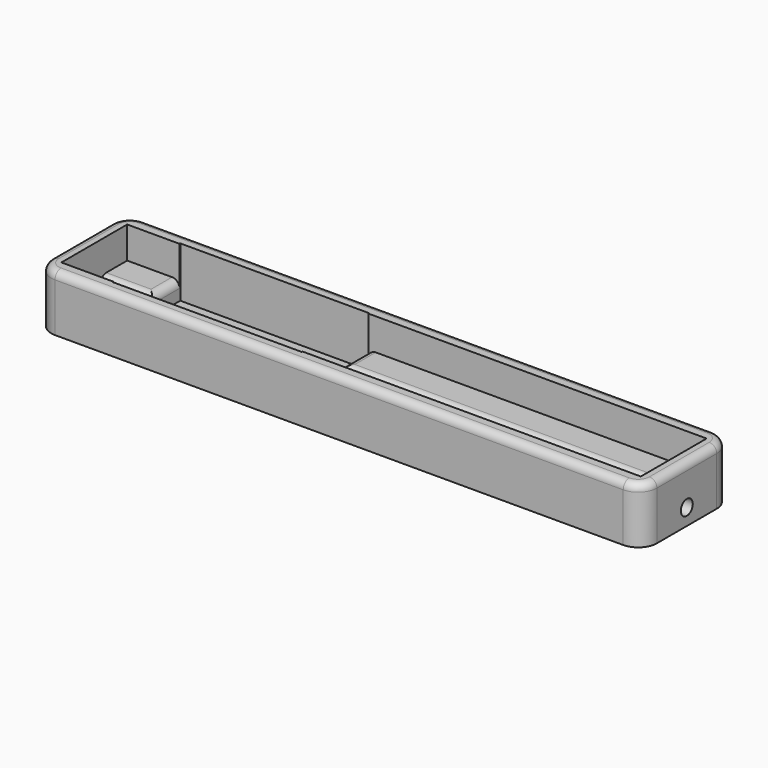
from build123d import *

# Parameters (mm, degrees)
F0_W         = 50.5
F0_H         = 9
F0_H_2       = 2
F0_W_2       = 12.75
F0_H_3       = 0.25
F0_W_3       = 1.2480659857
F1_DEPTH     = 1.5
F0_W_4       = 77.7519340143
F2_DEPTH     = 6.5
F3_DEPTH     = 15
F4_R         = 2
F5_DEPTH     = 162.001
F6_R         = 2
F7_T1_DEPTH  = 27.5
F7_T4_ANGLE  = 90
F7_T6_ANGLE  = 90
F7_T8_ANGLE  = 90
F7_T10_ANGLE = 90


# Not quite as in the source:
# - a fillet or chamfer that OpenCascade refuses, or shapes differently, is made with other operations: its cross-section is extruded or revolved along the edge and cut away or added


with BuildPart() as f1:
    # F0 (on Top) → F1 (new body)
    with BuildSketch(Plane.XY):
        with Locations((8.0849453807, 6.5)):
            Rectangle(F0_W, F0_H)
        with Locations((8.0849453807, 1)):
            Rectangle(F0_W, F0_H_2)
        with Locations((8.0849453807, -1)):
            Rectangle(F0_W, F0_H_2)
        with Locations((-23.5400546193, -1)):
            Rectangle(F0_W_2, F0_H_2)
        with Locations((-23.5400546193, 1)):
            Rectangle(F0_W_2, F0_H_2)
        with Locations((39.7099453807, 1)):
            Rectangle(F0_W_2, F0_H_2)
        with Locations((39.7099453807, -1)):
            Rectangle(F0_W_2, F0_H_2)
        Polygon((46.0849453807, 2), (46.0849453807, 0), (46.0849453807, -2), (123.8368793949, -2), (123.8368793949, 2), align=None)
        with Locations((8.0849453807, -6.5)):
            Rectangle(F0_W, F0_H)
        with Locations((8.0849453807, 11.125)):
            Rectangle(F0_W, F0_H_3)
        with Locations((8.0849453807, -11.125)):
            Rectangle(F0_W, F0_H_3)
        with Locations((-30.5390876122, -1)):
            Rectangle(F0_W_3, F0_H_2)
        with Locations((-30.5390876122, 1)):
            Rectangle(F0_W_3, F0_H_2)
    extrude(amount=F1_DEPTH)

    # F0 (on Top) → F2 (join)
    with BuildSketch(Plane.XY):
        with Locations((-23.5400546193, 6.5)):
            Rectangle(F0_W_2, F0_H)
        with Locations((-30.5390876122, 6.5)):
            Rectangle(F0_W_3, F0_H)
        with Locations((-23.5400546193, -6.5)):
            Rectangle(F0_W_2, F0_H)
        with Locations((-30.5390876122, -6.5)):
            Rectangle(F0_W_3, F0_H)
        with Locations((39.7099453807, -6.5)):
            Rectangle(F0_W_2, F0_H)
        with Locations((39.7099453807, 6.5)):
            Rectangle(F0_W_2, F0_H)
        with Locations((84.9609123878, 6.5)):
            Rectangle(F0_W_4, F0_H)
        with Locations((84.9609123878, -6.5)):
            Rectangle(F0_W_4, F0_H)
    extrude(amount=F2_DEPTH)

    # F0 (on Top) → F3 (join)
    with BuildSketch(Plane.XY):
        Polygon((127.3368793949, -15), (127.3368793949, 15), (-34.6631206051, 15), (-34.6631206051, 0), (-34.6631206051, -15), align=None)
        Polygon((-31.1631206051, -2), (-31.1631206051, 0), (-31.1631206051, 2), (-31.1631206051, 11), (-29.9150546193, 11), (-17.1650546193, 11), (-17.1650546193, 11.25), (33.3349453807, 11.25), (33.3349453807, 11), (46.0849453807, 11), (123.8368793949, 11), (123.8368793949, 2), (123.8368793949, -2), (123.8368793949, -11), (46.0849453807, -11), (33.3349453807, -11), (33.3349453807, -11.25), (-17.1650546193, -11.25), (-17.1650546193, -11), (-29.9150546193, -11), (-31.1631206051, -11), align=None, mode=Mode.SUBTRACT)
    extrude(amount=F3_DEPTH)

    # F4 (on face) → F5 (cut, through all)
    with BuildSketch(Plane.YZ.offset(127.3368793949)):
        with Locations((0, 4.3932246044)):
            Circle(F4_R)
    extrude(amount=-F5_DEPTH, mode=Mode.SUBTRACT)

    # F6
    f6_edges = [f1.edges().sort_by_distance(p)[0] for p in [
        (-24.164088, -2, 6.5),
        (-24.164088, 2, 6.5),
        (-17.165055, -6.5, 6.5),
        (-17.165055, 6.5, 6.5),
        (33.334945, 6.5, 6.5),
        (33.334945, -6.5, 6.5),
        (78.585912, -2, 6.5),
        (78.585912, 2, 6.5),
        (46.336879, 15, 15),
        (-34.663121, 0, 15),
        (46.336879, -15, 15),
        (127.336879, 0, 15),
    ]]
    fillet(f6_edges, radius=F6_R)

    # F7: fillet of radius 5 on 4 edges, made by hand

    # F7_s2 → F7_t1 (cut)
    with BuildSketch(Plane.XY.offset(-12.5)):
        with BuildLine():
            ThreePointArc((-29.6631206051, 15), (-33.198654511, 13.5355339059), (-34.6631206051, 10))
            Line((-34.6631206051, 10), (-34.6631206051, 15))
            Line((-34.6631206051, 15), (-29.6631206051, 15))
        make_face()
        with BuildLine():
            ThreePointArc((-34.6631206051, -10), (-33.198654511, -13.5355339059), (-29.6631206051, -15))
            Line((-29.6631206051, -15), (-34.6631206051, -15))
            Line((-34.6631206051, -15), (-34.6631206051, -10))
        make_face()
        with BuildLine():
            ThreePointArc((122.3368793949, 15), (125.8724133009, 13.5355339059), (127.3368793949, 10))
            Line((127.3368793949, 10), (127.3368793949, 15))
            Line((127.3368793949, 15), (122.3368793949, 15))
        make_face()
        with BuildLine():
            ThreePointArc((127.3368793949, -10), (125.8724133009, -13.5355339059), (122.3368793949, -15))
            Line((122.3368793949, -15), (127.3368793949, -15))
            Line((127.3368793949, -15), (127.3368793949, -10))
        make_face()
    extrude(amount=F7_T1_DEPTH, mode=Mode.SUBTRACT)

    # F7_s3 → F7_t4 (revolve, cut)
    with BuildSketch(Plane.YZ.offset(122.3368793949)):
        with BuildLine():
            ThreePointArc((-13, 15), (-14.4142135624, 14.4142135624), (-15, 13))
            Line((-15, 13), (-15, 15))
            Line((-15, 15), (-13, 15))
        make_face()
    revolve(axis=Axis((122.3368793949, -10, 15), (0, 0, 1)), revolution_arc=F7_T4_ANGLE, mode=Mode.SUBTRACT)

    # F7_s5 → F7_t6 (revolve, cut)
    with BuildSketch(Plane.XZ.offset(-10)):
        with BuildLine():
            ThreePointArc((125.3368793949, 15), (126.7510929573, 14.4142135624), (127.3368793949, 13))
            Line((127.3368793949, 13), (127.3368793949, 15))
            Line((127.3368793949, 15), (125.3368793949, 15))
        make_face()
    revolve(axis=Axis((122.3368793949, 10, 15), (0, 0, 1)), revolution_arc=F7_T6_ANGLE, mode=Mode.SUBTRACT)

    # F7_s7 → F7_t8 (revolve, cut)
    with BuildSketch(Plane.XZ.offset(10)):
        with BuildLine():
            ThreePointArc((-32.6631206051, 15), (-34.0773341674, 14.4142135624), (-34.6631206051, 13))
            Line((-34.6631206051, 13), (-34.6631206051, 15))
            Line((-34.6631206051, 15), (-32.6631206051, 15))
        make_face()
    revolve(axis=Axis((-29.6631206051, -10, 15), (0, 0, 1)), revolution_arc=F7_T8_ANGLE, mode=Mode.SUBTRACT)

    # F7_s9 → F7_t10 (revolve, cut)
    with BuildSketch(Plane.YZ.offset(-29.6631206051)):
        with BuildLine():
            ThreePointArc((13, 15), (14.4142135624, 14.4142135624), (15, 13))
            Line((15, 13), (15, 15))
            Line((15, 15), (13, 15))
        make_face()
    revolve(axis=Axis((-29.6631206051, 10, 15), (0, 0, 1)), revolution_arc=F7_T10_ANGLE, mode=Mode.SUBTRACT)


solid = f1.part
